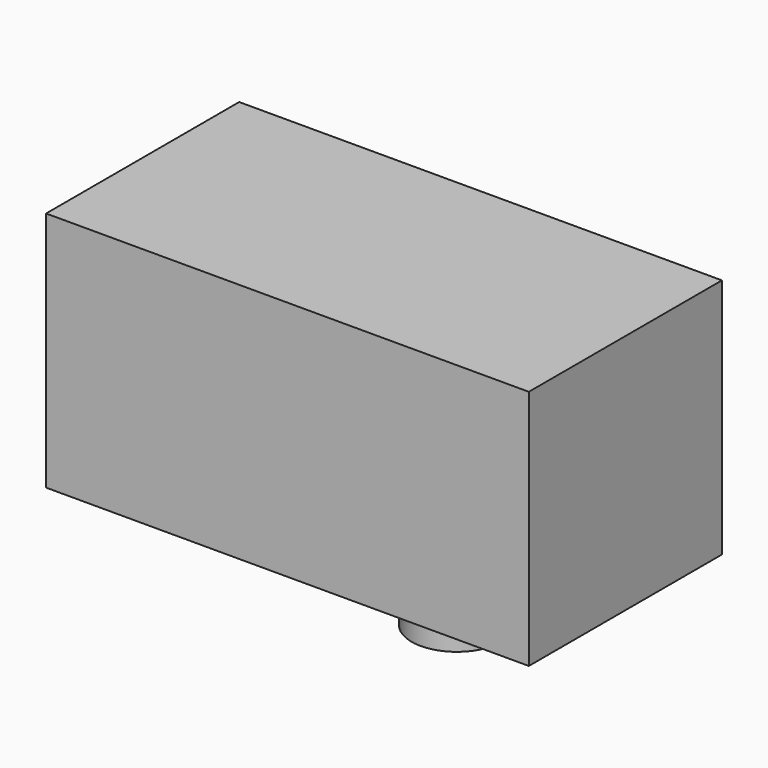
from build123d import *

# Parameters (mm, degrees)
F0_W      = 406.4
F0_H      = 203.2
F1_DEPTH  = 101.6
F4_W      = 393.7
F4_H      = 190.5
F5_DEPTH  = 190.5
F6_R      = 38.1
F7_DEPTH  = 6.35
F10_DEPTH = 101.6


# Not quite as in the source:
# - the program builds the solid bodies; features that only make, move or delete a surface that nothing else refers to are left out


with BuildPart() as f1:
    # F0 (on Top) → F1 (new body, symmetric)
    with BuildSketch(Plane.XY):
        with Locations((-1.672681421, -62.5133958211)):
            Rectangle(F0_W, F0_H)
    extrude(amount=F1_DEPTH, both=True)

    # F4 (on offset) → F5 (cut)
    with BuildSketch(Plane.XZ.offset(157.7633958211)):
        with Locations((-1.672681421, 0)):
            Rectangle(F4_W, F4_H)
    extrude(amount=-F5_DEPTH, mode=Mode.SUBTRACT)

    # F6 (on face) → F7 (cut, through all)
    with BuildSketch(Plane(origin=(0, 0, -101.6), x_dir=(1, 0, 0), z_dir=(0, 0, -1))):
        with Locations((13.9572741464, 5.3633958211)):
            Circle(F6_R)
    extrude(amount=-F7_DEPTH, mode=Mode.SUBTRACT)

    # F9 (on offset) → F10 (join)
    with BuildSketch(Plane(origin=(0, 0, -95.25), x_dir=(1, 0, 0), z_dir=(0, 0, -1))):
        with BuildLine():
            ThreePointArc((13.9572742307, -32.7366041789), (40.8980425394, -21.5773725123), (52.0572741464, 5.3633958211))
            ThreePointArc((52.0572741464, 5.3633958211), (-12.9834942466, 32.3041641545), (13.9572742307, -32.7366041789))
        make_face()
    extrude(amount=F10_DEPTH)


solid = f1.part
